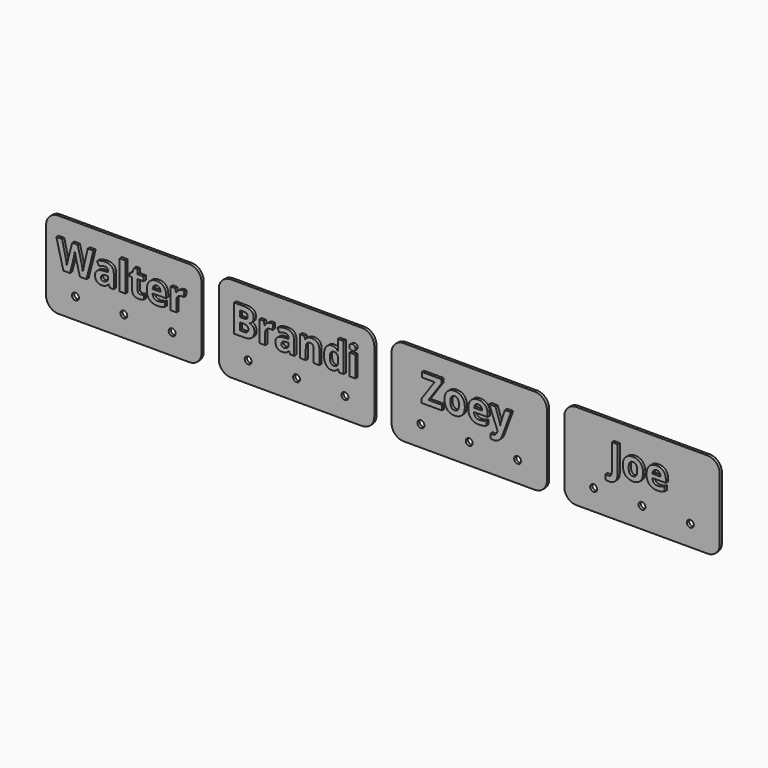
from build123d import *

# Parameters (mm, degrees)
F0_R         = 2
F1_DEPTH     = 1.6
F2_TEXT_SIZE = 22.2222222222
F3_DEPTH     = 1.6
F4_TEXT_SIZE = 22.2222222222
F5_DEPTH     = 1.6
F6_TEXT_SIZE = 22.2222222222
F7_DEPTH     = 1.6
F8_TEXT_SIZE = 22.2222222222
F9_DEPTH     = 1.6


# Not quite as in the source:
# - Text() gives the source's letters only with a copy of the font that has no kerning and outlines rounded to 1/6400 em; it was checked with that copy


with BuildPart() as f1:
    # F0 (on Front) → F1 (new body)
    with BuildSketch(Plane.XZ):
        with BuildLine():
            ThreePointArc((71.9894273281, 48.3366710152), (67.0396798598, 46.2864184836), (64.9894273281, 41.3366710152))
            Line((64.9894273281, 41.3366710152), (64.9894273281, 5.3366710152))
            ThreePointArc((64.9894273281, 5.3366710152), (67.0396798598, 0.3869235469), (71.9894273281, -1.6633289848))
            Line((71.9894273281, -1.6633289848), (147.9894273281, -1.6633289848))
            ThreePointArc((147.9894273281, -1.6633289848), (152.9391747964, 0.3869235469), (154.9894273281, 5.3366710152))
            Line((154.9894273281, 5.3366710152), (154.9894273281, 41.3366710152))
            ThreePointArc((154.9894273281, 41.3366710152), (152.9391747964, 46.2864184836), (147.9894273281, 48.3366710152))
            Line((147.9894273281, 48.3366710152), (71.9894273281, 48.3366710152))
        make_face()
        with Locations((81.9894273281, 10.3366710152)):
            Circle(F0_R, mode=Mode.SUBTRACT)
        with Locations((109.9894273281, 10.3366710152)):
            Circle(F0_R, mode=Mode.SUBTRACT)
        with Locations((137.9894273281, 10.3366710152)):
            Circle(F0_R, mode=Mode.SUBTRACT)
    extrude(amount=-F1_DEPTH)

    # F4 (on face) → F5 (join)
    with BuildSketch(Plane.XZ):
        with Locations((73.1144273281, 22.3366710152)):
            Text('Brandi', F4_TEXT_SIZE, font='Open Sans', font_style=FontStyle.BOLD, text_align=(TextAlign.LEFT, TextAlign.BOTTOM))
    extrude(amount=F5_DEPTH)


with BuildPart() as f1b:
    # F0 (on Front) → F1, piece 2 (new body)
    with BuildSketch(Plane.XZ):
        with BuildLine():
            ThreePointArc((171.9894273281, 48.3366710152), (167.0396798598, 46.2864184836), (164.9894273281, 41.3366710152))
            Line((164.9894273281, 41.3366710152), (164.9894273281, 5.3366710152))
            ThreePointArc((164.9894273281, 5.3366710152), (167.0396798598, 0.3869235469), (171.9894273281, -1.6633289848))
            Line((171.9894273281, -1.6633289848), (247.9894273281, -1.6633289848))
            ThreePointArc((247.9894273281, -1.6633289848), (252.9391747964, 0.3869235469), (254.9894273281, 5.3366710152))
            Line((254.9894273281, 5.3366710152), (254.9894273281, 41.3366710152))
            ThreePointArc((254.9894273281, 41.3366710152), (252.9391747964, 46.2864184836), (247.9894273281, 48.3366710152))
            Line((247.9894273281, 48.3366710152), (171.9894273281, 48.3366710152))
        make_face()
        with Locations((181.9894273281, 10.3366710152)):
            Circle(F0_R, mode=Mode.SUBTRACT)
        with Locations((209.9894273281, 10.3366710152)):
            Circle(F0_R, mode=Mode.SUBTRACT)
        with Locations((237.9894273281, 10.3366710152)):
            Circle(F0_R, mode=Mode.SUBTRACT)
    extrude(amount=-F1_DEPTH)

    # F6 (on face) → F7 (join)
    with BuildSketch(Plane.XZ):
        with Locations((183.0692884392, 22.3366710152)):
            Text('Zoey', F6_TEXT_SIZE, font='Open Sans', font_style=FontStyle.BOLD, text_align=(TextAlign.LEFT, TextAlign.BOTTOM))
    extrude(amount=F7_DEPTH)


with BuildPart() as f1c:
    # F0 (on Front) → F1, piece 3 (new body)
    with BuildSketch(Plane.XZ):
        with BuildLine():
            Line((47.9894273281, 48.3366710152), (-28.0105726719, 48.3366710152))
            ThreePointArc((-28.0105726719, 48.3366710152), (-32.9603201402, 46.2864184836), (-35.0105726719, 41.3366710152))
            Line((-35.0105726719, 41.3366710152), (-35.0105726719, 5.3366710152))
            ThreePointArc((-35.0105726719, 5.3366710152), (-32.9603201402, 0.3869235469), (-28.0105726719, -1.6633289848))
            Line((-28.0105726719, -1.6633289848), (47.9894273281, -1.6633289848))
            ThreePointArc((47.9894273281, -1.6633289848), (52.9391747964, 0.3869235469), (54.9894273281, 5.3366710152))
            Line((54.9894273281, 5.3366710152), (54.9894273281, 41.3366710152))
            ThreePointArc((54.9894273281, 41.3366710152), (52.9391747964, 46.2864184836), (47.9894273281, 48.3366710152))
        make_face()
        with Locations((-18.0105726719, 10.3366710152)):
            Circle(F0_R, mode=Mode.SUBTRACT)
        with Locations((9.9894273281, 10.3366710152)):
            Circle(F0_R, mode=Mode.SUBTRACT)
        with Locations((37.9894273281, 10.3366710152)):
            Circle(F0_R, mode=Mode.SUBTRACT)
    extrude(amount=-F1_DEPTH)

    # F2 (on face) → F3 (join)
    with BuildSketch(Plane.XZ):
        with Locations((-27.7761976719, 22.3366710152)):
            Text('Walter', F2_TEXT_SIZE, font='Open Sans', font_style=FontStyle.BOLD, text_align=(TextAlign.LEFT, TextAlign.BOTTOM))
    extrude(amount=F3_DEPTH)


with BuildPart() as f1d:
    # F0 (on Front) → F1, piece 4 (new body)
    with BuildSketch(Plane.XZ):
        with BuildLine():
            ThreePointArc((271.9894273281, 48.3366710152), (267.0396798598, 46.2864184836), (264.9894273281, 41.3366710152))
            Line((264.9894273281, 41.3366710152), (264.9894273281, 5.3366710152))
            ThreePointArc((264.9894273281, 5.3366710152), (267.0396798598, 0.3869235469), (271.9894273281, -1.6633289848))
            Line((271.9894273281, -1.6633289848), (347.9894273281, -1.6633289848))
            ThreePointArc((347.9894273281, -1.6633289848), (352.9391747964, 0.3869235469), (354.9894273281, 5.3366710152))
            Line((354.9894273281, 5.3366710152), (354.9894273281, 41.3366710152))
            ThreePointArc((354.9894273281, 41.3366710152), (352.9391747964, 46.2864184836), (347.9894273281, 48.3366710152))
            Line((347.9894273281, 48.3366710152), (271.9894273281, 48.3366710152))
        make_face()
        with Locations((281.9894273281, 10.3366710152)):
            Circle(F0_R, mode=Mode.SUBTRACT)
        with Locations((309.9894273281, 10.3366710152)):
            Circle(F0_R, mode=Mode.SUBTRACT)
        with Locations((337.9894273281, 10.3366710152)):
            Circle(F0_R, mode=Mode.SUBTRACT)
    extrude(amount=-F1_DEPTH)

    # F8 (on face) → F9 (join)
    with BuildSketch(Plane.XZ):
        with Locations((291.7984551059, 22.3366710152)):
            Text('Joe', F8_TEXT_SIZE, font='Open Sans', font_style=FontStyle.BOLD, text_align=(TextAlign.LEFT, TextAlign.BOTTOM))
    extrude(amount=F9_DEPTH)


solid = Compound([f1.part, f1b.part, f1c.part, f1d.part])
